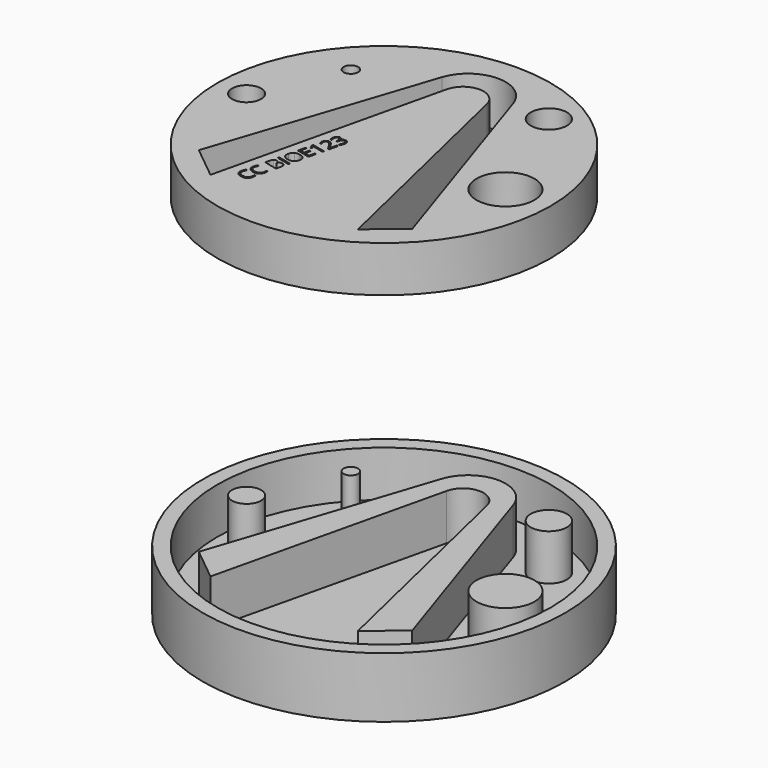
from build123d import *

# Parameters (mm, degrees)
F0_R     = 23
F1_DEPTH = 2
F3_R     = 2
F3_R_2   = 4
F3_R_3   = 1
F3_R_4   = 2.5
F4_DEPTH = 6.35
F0_R_2   = 25
F5_DEPTH = 8.35
F6_R     = 23
F6_R_2   = 2
F6_R_3   = 1
F6_R_4   = 4
F6_R_5   = 2.5
F7_DEPTH = 6.35


# Not quite as in the source:
# - a feature names something its author has since deleted; it is built from what else it names


with BuildPart() as f1:
    # F0 (on Top) → F1 (new body)
    with BuildSketch(Plane.XY):
        Circle(F0_R)
    extrude(amount=F1_DEPTH)

    # F3 (on face) → F4 (join)
    with BuildSketch(Plane.XY.offset(2)):
        with BuildLine():
            Line((14.693104138, -13.4988571827), (4.888704138, 16.1648631611))
            ThreePointArc((4.888704138, 16.1648631611), (-0.032147931, 19.721101458), (-4.953, 16.1648631611))
            Line((-4.953, 16.1648631611), (-14.7574, -13.4988571827))
            Line((-14.7574, -13.4988571827), (-10.182928455, -17.2135983478))
            Line((-10.182928455, -17.2135983478), (-2.7686, 14.2851547342))
            ThreePointArc((-2.7686, 14.2851547342), (-0.0045905534, 16.4740974526), (2.7594188933, 14.2851547342))
            Line((2.7594188933, 14.2851547342), (10.1737473482, -17.2135983478))
            Line((10.1737473482, -17.2135983478), (14.693104138, -13.4988571827))
        make_face()
        with Locations((-18.9738, 0)):
            Circle(F3_R)
        with Locations((16.764, 0)):
            Circle(F3_R_2)
        with Locations((-13.716, 11.43)):
            Circle(F3_R_3)
        with Locations((10.16, 15.748)):
            Circle(F3_R_4)
    extrude(amount=F4_DEPTH)

    # F0 (on Top) → F5 (join)
    with BuildSketch(Plane.XY):
        Circle(F0_R_2)
        Circle(F0_R, mode=Mode.SUBTRACT)
    extrude(amount=F5_DEPTH)


with BuildPart() as f7:
    # F6 (on offset) → F7 (new body)
    with BuildSketch(Plane.XY.offset(50.8)):
        Circle(F6_R)
        with BuildLine():
            add(Edge.make_bspline(
                [(-7.7742172335, -13.9858252735), (-7.9195629499, -14.1696054685), (-7.9681992906, -14.3761575918)],
                knots=[0, 0, 0, 1, 1, 1], degree=2))
            add(Edge.make_bspline(
                [(-7.9681992906, -14.3761575918), (-8.038764155, -14.6758372619), (-7.8800349733, -14.8963533518)],
                knots=[0, 0, 0, 1, 1, 1], degree=2))
            add(Edge.make_bspline(
                [(-7.8800349733, -14.8963533518), (-7.7213057917, -15.1168694417), (-7.3742663861, -15.198585991)],
                knots=[0, 0, 0, 1, 1, 1], degree=2))
            add(Edge.make_bspline(
                [(-7.3742663861, -15.198585991), (-7.0176754372, -15.2825516198), (-6.7834580083, -15.1610724694)],
                knots=[0, 0, 0, 1, 1, 1], degree=2))
            add(Edge.make_bspline(
                [(-6.7834580083, -15.1610724694), (-6.5492405793, -15.039593319), (-6.476332924, -14.7299641245)],
                knots=[0, 0, 0, 1, 1, 1], degree=2))
            add(Edge.make_bspline(
                [(-6.476332924, -14.7299641245), (-6.4315387605, -14.539729221), (-6.4425462525, -14.2796484846)],
                knots=[0, 0, 0, 1, 1, 1], degree=2))
            Line((-6.4425462525, -14.2796484846), (-6.2574851015, -14.3232243969))
            add(Edge.make_bspline(
                [(-6.2574851015, -14.3232243969), (-6.2307595366, -14.5290397409), (-6.2960765491, -14.8064324768)],
                knots=[0, 0, 0, 1, 1, 1], degree=2))
            add(Edge.make_bspline(
                [(-6.2960765491, -14.8064324768), (-6.390631593, -15.2079952752), (-6.6859947616, -15.3688426023)],
                knots=[0, 0, 0, 1, 1, 1], degree=2))
            add(Edge.make_bspline(
                [(-6.6859947616, -15.3688426023), (-6.9813579301, -15.5296899294), (-7.430280464, -15.4239832004)],
                knots=[0, 0, 0, 1, 1, 1], degree=2))
            add(Edge.make_bspline(
                [(-7.430280464, -15.4239832004), (-7.7112550286, -15.3578227831), (-7.8978430508, -15.2029949267)],
                knots=[0, 0, 0, 1, 1, 1], degree=2))
            add(Edge.make_bspline(
                [(-7.8978430508, -15.2029949267), (-8.0844310729, -15.0481670703), (-8.1521353496, -14.8228314606)],
                knots=[0, 0, 0, 1, 1, 1], degree=2))
            add(Edge.make_bspline(
                [(-8.1521353496, -14.8228314606), (-8.2198396262, -14.5974958509), (-8.1565842698, -14.3288586963)],
                knots=[0, 0, 0, 1, 1, 1], degree=2))
            add(Edge.make_bspline(
                [(-8.1565842698, -14.3288586963), (-8.0892993128, -14.0431083601), (-7.9346114369, -13.8535470478)],
                knots=[0, 0, 0, 1, 1, 1], degree=2))
            Line((-7.9346114369, -13.8535470478), (-7.7742172335, -13.9858252735))
        make_face(mode=Mode.SUBTRACT)
        with BuildLine():
            add(Edge.make_bspline(
                [(-7.3958096344, -12.3787781178), (-7.5411553508, -12.5625583127), (-7.5897916916, -12.769110436)],
                knots=[0, 0, 0, 1, 1, 1], degree=2))
            add(Edge.make_bspline(
                [(-7.5897916916, -12.769110436), (-7.6603565559, -13.0687901062), (-7.5016273743, -13.2893061961)],
                knots=[0, 0, 0, 1, 1, 1], degree=2))
            add(Edge.make_bspline(
                [(-7.5016273743, -13.2893061961), (-7.3428981926, -13.5098222859), (-6.995858787, -13.5915388353)],
                knots=[0, 0, 0, 1, 1, 1], degree=2))
            add(Edge.make_bspline(
                [(-6.995858787, -13.5915388353), (-6.6392678382, -13.675504464), (-6.4050504092, -13.5540253136)],
                knots=[0, 0, 0, 1, 1, 1], degree=2))
            add(Edge.make_bspline(
                [(-6.4050504092, -13.5540253136), (-6.1708329803, -13.4325461633), (-6.097925325, -13.1229169688)],
                knots=[0, 0, 0, 1, 1, 1], degree=2))
            add(Edge.make_bspline(
                [(-6.097925325, -13.1229169688), (-6.0531311614, -12.9326820653), (-6.0641386534, -12.6726013289)],
                knots=[0, 0, 0, 1, 1, 1], degree=2))
            Line((-6.0641386534, -12.6726013289), (-5.8790775025, -12.7161772411))
            add(Edge.make_bspline(
                [(-5.8790775025, -12.7161772411), (-5.8523519375, -12.9219925852), (-5.91766895, -13.1993853211)],
                knots=[0, 0, 0, 1, 1, 1], degree=2))
            add(Edge.make_bspline(
                [(-5.91766895, -13.1993853211), (-6.012223994, -13.6009481195), (-6.3075871625, -13.7617954466)],
                knots=[0, 0, 0, 1, 1, 1], degree=2))
            add(Edge.make_bspline(
                [(-6.3075871625, -13.7617954466), (-6.602950331, -13.9226427736), (-7.0518728649, -13.8169360446)],
                knots=[0, 0, 0, 1, 1, 1], degree=2))
            add(Edge.make_bspline(
                [(-7.0518728649, -13.8169360446), (-7.3328474295, -13.7507756274), (-7.5194354517, -13.5959477709)],
                knots=[0, 0, 0, 1, 1, 1], degree=2))
            add(Edge.make_bspline(
                [(-7.5194354517, -13.5959477709), (-7.7060234739, -13.4411199145), (-7.7737277505, -13.2157843049)],
                knots=[0, 0, 0, 1, 1, 1], degree=2))
            add(Edge.make_bspline(
                [(-7.7737277505, -13.2157843049), (-7.8414320272, -12.9904486952), (-7.7781766707, -12.7218115406)],
                knots=[0, 0, 0, 1, 1, 1], degree=2))
            add(Edge.make_bspline(
                [(-7.7781766707, -12.7218115406), (-7.7108917138, -12.4360612044), (-7.5562038378, -12.2464998921)],
                knots=[0, 0, 0, 1, 1, 1], degree=2))
            Line((-7.5562038378, -12.2464998921), (-7.3958096344, -12.3787781178))
        make_face(mode=Mode.SUBTRACT)
        with BuildLine():
            Line((-5.5836387497, -11.6684184118), (-7.4020138004, -11.2402499324))
            Line((-7.4020138004, -11.2402499324), (-7.2810320742, -10.7264565005))
            add(Edge.make_bspline(
                [(-7.2810320742, -10.7264565005), (-7.1958481942, -10.364691799), (-7.0495035891, -10.2284021007)],
                knots=[0, 0, 0, 1, 1, 1], degree=2))
            add(Edge.make_bspline(
                [(-7.0495035891, -10.2284021007), (-6.903158984, -10.0921124023), (-6.6695441547, -10.1471211345)],
                knots=[0, 0, 0, 1, 1, 1], degree=2))
            add(Edge.make_bspline(
                [(-6.6695441547, -10.1471211345), (-6.5075659001, -10.1852617717), (-6.4237246103, -10.3001443341)],
                knots=[0, 0, 0, 1, 1, 1], degree=2))
            add(Edge.make_bspline(
                [(-6.4237246103, -10.3001443341), (-6.3398833206, -10.4150268965), (-6.349605368, -10.5954581261)],
                knots=[0, 0, 0, 1, 1, 1], degree=2))
            Line((-6.349605368, -10.5954581261), (-6.337267958, -10.598363187))
            add(Edge.make_bspline(
                [(-6.337267958, -10.598363187), (-6.1688735289, -10.2007456693), (-5.8043229607, -10.2865855308)],
                knots=[0, 0, 0, 1, 1, 1], degree=2))
            add(Edge.make_bspline(
                [(-5.8043229607, -10.2865855308), (-5.5607586072, -10.3439370539), (-5.4626497723, -10.5409379793)],
                knots=[0, 0, 0, 1, 1, 1], degree=2))
            add(Edge.make_bspline(
                [(-5.4626497723, -10.5409379793), (-5.3645409373, -10.7379389046), (-5.4342623969, -11.0340367461)],
                knots=[0, 0, 0, 1, 1, 1], degree=2))
            Line((-5.4342623969, -11.0340367461), (-5.5836387497, -11.6684184118))
        make_face(mode=Mode.SUBTRACT)
        Polygon((-5.1452557016, -9.8066634355), (-5.195016582, -10.0179913304), (-7.0133916326, -9.5898228509), (-6.9636307522, -9.378494956), align=None, mode=Mode.SUBTRACT)
        with BuildLine():
            add(Edge.make_bspline(
                [(-6.3062887675, -7.5733382878), (-6.0057281249, -7.411824586), (-5.5679490583, -7.5149073891)],
                knots=[0, 0, 0, 1, 1, 1], degree=2))
            add(Edge.make_bspline(
                [(-5.5679490583, -7.5149073891), (-5.1313639345, -7.6177090573), (-4.9332428548, -7.8974862608)],
                knots=[0, 0, 0, 1, 1, 1], degree=2))
            add(Edge.make_bspline(
                [(-4.9332428548, -7.8974862608), (-4.735121775, -8.1772634642), (-4.8276151629, -8.5700706813)],
                knots=[0, 0, 0, 1, 1, 1], degree=2))
            add(Edge.make_bspline(
                [(-4.8276151629, -8.5700706813), (-4.9221702069, -8.9716334798), (-5.2193242898, -9.1320591044)],
                knots=[0, 0, 0, 1, 1, 1], degree=2))
            add(Edge.make_bspline(
                [(-5.2193242898, -9.1320591044), (-5.5164783727, -9.2924847291), (-5.9642069636, -9.187059135)],
                knots=[0, 0, 0, 1, 1, 1], degree=2))
            add(Edge.make_bspline(
                [(-5.9642069636, -9.187059135), (-6.4083537258, -9.0824769457), (-6.6011726397, -8.8060484659)],
                knots=[0, 0, 0, 1, 1, 1], degree=2))
            add(Edge.make_bspline(
                [(-6.6011726397, -8.8060484659), (-6.7939915535, -8.5296199861), (-6.6991553747, -8.1268632447)],
                knots=[0, 0, 0, 1, 1, 1], degree=2))
            add(Edge.make_bspline(
                [(-6.6991553747, -8.1268632447), (-6.60684941, -7.7348519895), (-6.3062887675, -7.5733382878)],
                knots=[0, 0, 0, 1, 1, 1], degree=2))
        make_face(mode=Mode.SUBTRACT)
        Polygon((-4.5111336235, -6.2662855689), (-4.3220926629, -6.3107985975), (-4.5607762079, -7.3244561274), (-6.3791512586, -6.8962876479), (-6.1404677136, -5.882630118), (-5.9526206958, -5.9268620117), (-6.1415433605, -6.7291916467), (-5.555715373, -6.8671351796), (-5.3782255284, -6.1133592229), (-5.1915724536, -6.1573099817), (-5.3690622982, -6.9110859383), (-4.7000562881, -7.0686152038), align=None, mode=Mode.SUBTRACT)
        with BuildLine():
            Line((-5.8951306421, -4.8407159393), (-4.0767555915, -5.2688844188))
            Line((-4.0767555915, -5.2688844188), (-4.1241736809, -5.4702627894))
            Line((-4.1241736809, -5.4702627894), (-5.4199997183, -5.1651376922))
            add(Edge.make_bspline(
                [(-5.4199997183, -5.1651376922), (-5.581977973, -5.1269970551), (-5.7237042931, -5.0831239174)],
                knots=[0, 0, 0, 1, 1, 1], degree=2))
            add(Edge.make_bspline(
                [(-5.7237042931, -5.0831239174), (-5.7035288056, -5.1151776487), (-5.6827106649, -5.1543134799)],
                knots=[0, 0, 0, 1, 1, 1], degree=2))
            add(Edge.make_bspline(
                [(-5.6827106649, -5.1543134799), (-5.6618925241, -5.1934493111), (-5.5098158676, -5.507329575)],
                knots=[0, 0, 0, 1, 1, 1], degree=2))
            Line((-5.5098158676, -5.507329575), (-5.6772677936, -5.5834129981))
            Line((-5.6772677936, -5.5834129981), (-5.9360826285, -5.0146336231))
            Line((-5.9360826285, -5.0146336231), (-5.8951306421, -4.8407159393))
        make_face(mode=Mode.SUBTRACT)
        with BuildLine():
            Line((-3.8238975565, -3.3369813429), (-3.6324687101, -3.3820566413))
            Line((-3.6324687101, -3.3820566413), (-3.9138847626, -4.5771934934))
            Line((-3.9138847626, -4.5771934934), (-4.091782256, -4.5353043907))
            Line((-4.091782256, -4.5353043907), (-4.4602061465, -3.9432359123))
            add(Edge.make_bspline(
                [(-4.4602061465, -3.9432359123), (-4.6303401451, -3.6721489959), (-4.7084610885, -3.5802458119)],
                knots=[0, 0, 0, 1, 1, 1], degree=2))
            add(Edge.make_bspline(
                [(-4.7084610885, -3.5802458119), (-4.786582032, -3.4883426279), (-4.8679279817, -3.4324341743)],
                knots=[0, 0, 0, 1, 1, 1], degree=2))
            add(Edge.make_bspline(
                [(-4.8679279817, -3.4324341743), (-4.9492739315, -3.3765257206), (-5.0523510026, -3.352254406)],
                knots=[0, 0, 0, 1, 1, 1], degree=2))
            add(Edge.make_bspline(
                [(-5.0523510026, -3.352254406), (-5.1980120375, -3.3179559461), (-5.303983949, -3.3862534306)],
                knots=[0, 0, 0, 1, 1, 1], degree=2))
            add(Edge.make_bspline(
                [(-5.303983949, -3.3862534306), (-5.4099558604, -3.4545509151), (-5.4468782462, -3.6113554171)],
                knots=[0, 0, 0, 1, 1, 1], degree=2))
            add(Edge.make_bspline(
                [(-5.4468782462, -3.6113554171), (-5.4734923518, -3.7243820125), (-5.4599786086, -3.8346760539)],
                knots=[0, 0, 0, 1, 1, 1], degree=2))
            add(Edge.make_bspline(
                [(-5.4599786086, -3.8346760539), (-5.4464648654, -3.9449700953), (-5.3774015974, -4.0922869327)],
                knots=[0, 0, 0, 1, 1, 1], degree=2))
            Line((-5.3774015974, -4.0922869327), (-5.5436595804, -4.1686514907))
            add(Edge.make_bspline(
                [(-5.5436595804, -4.1686514907), (-5.6934675452, -3.8683268883), (-5.6237460857, -3.5722290468)],
                knots=[0, 0, 0, 1, 1, 1], degree=2))
            add(Edge.make_bspline(
                [(-5.6237460857, -3.5722290468), (-5.56339579, -3.3159293023), (-5.3980094564, -3.201345243)],
                knots=[0, 0, 0, 1, 1, 1], degree=2))
            add(Edge.make_bspline(
                [(-5.3980094564, -3.201345243), (-5.2326231227, -3.0867611837), (-5.0113457036, -3.1388648551)],
                knots=[0, 0, 0, 1, 1, 1], degree=2))
            add(Edge.make_bspline(
                [(-5.0113457036, -3.1388648551), (-4.8382239817, -3.1796294181), (-4.6919477096, -3.3165642214)],
                knots=[0, 0, 0, 1, 1, 1], degree=2))
            add(Edge.make_bspline(
                [(-4.6919477096, -3.3165642214), (-4.5456714374, -3.4534990246), (-4.3495831821, -3.7802628779)],
                knots=[0, 0, 0, 1, 1, 1], degree=2))
            Line((-4.3495831821, -3.7802628779), (-4.0540694329, -4.2698938307))
            Line((-4.0540694329, -4.2698938307), (-4.0441199086, -4.2722366217))
            Line((-4.0441199086, -4.2722366217), (-3.8238975565, -3.3369813429))
        make_face(mode=Mode.SUBTRACT)
        with BuildLine():
            add(Edge.make_bspline(
                [(-5.0633344275, -1.7354274359), (-4.9075696273, -1.6171076522), (-4.6962417324, -1.6668685326)],
                knots=[0, 0, 0, 1, 1, 1], degree=2))
            add(Edge.make_bspline(
                [(-4.6962417324, -1.6668685326), (-4.5219260677, -1.7079142305), (-4.4342935655, -1.8316703943)],
                knots=[0, 0, 0, 1, 1, 1], degree=2))
            add(Edge.make_bspline(
                [(-4.4342935655, -1.8316703943), (-4.3466610634, -1.9554265581), (-4.3514210898, -2.1433268885)],
                knots=[0, 0, 0, 1, 1, 1], degree=2))
            Line((-4.3514210898, -2.1433268885), (-4.3414715656, -2.1456696795))
            add(Edge.make_bspline(
                [(-4.3414715656, -2.1456696795), (-4.2628674581, -1.9331525376), (-4.1259553749, -1.8538684166)],
                knots=[0, 0, 0, 1, 1, 1], degree=2))
            add(Edge.make_bspline(
                [(-4.1259553749, -1.8538684166), (-3.9890432917, -1.7745842956), (-3.8075639695, -1.817316803)],
                knots=[0, 0, 0, 1, 1, 1], degree=2))
            add(Edge.make_bspline(
                [(-3.8075639695, -1.817316803), (-3.5476823963, -1.8785105034), (-3.4500444675, -2.0917823797)],
                knots=[0, 0, 0, 1, 1, 1], degree=2))
            add(Edge.make_bspline(
                [(-3.4500444675, -2.0917823797), (-3.3524065387, -2.305054256), (-3.4305620458, -2.6369703847)],
                knots=[0, 0, 0, 1, 1, 1], degree=2))
            add(Edge.make_bspline(
                [(-3.4305620458, -2.6369703847), (-3.4645793709, -2.7814374767), (-3.5147223834, -2.896274599)],
                knots=[0, 0, 0, 1, 1, 1], degree=2))
            add(Edge.make_bspline(
                [(-3.5147223834, -2.896274599), (-3.564865396, -3.0111117212), (-3.6460028943, -3.111299822)],
                knots=[0, 0, 0, 1, 1, 1], degree=2))
            Line((-3.6460028943, -3.111299822), (-3.8426054934, -3.0650062722))
            add(Edge.make_bspline(
                [(-3.8426054934, -3.0650062722), (-3.756269934, -2.9605815352), (-3.694337279, -2.8340288698)],
                knots=[0, 0, 0, 1, 1, 1], degree=2))
            add(Edge.make_bspline(
                [(-3.694337279, -2.8340288698), (-3.6324046241, -2.7074762043), (-3.6042911323, -2.5880819134)],
                knots=[0, 0, 0, 1, 1, 1], degree=2))
            add(Edge.make_bspline(
                [(-3.6042911323, -2.5880819134), (-3.4933365515, -2.1168724453), (-3.8626628914, -2.0299080441)],
                knots=[0, 0, 0, 1, 1, 1], degree=2))
            add(Edge.make_bspline(
                [(-3.8626628914, -2.0299080441), (-4.1937830582, -1.9519399603), (-4.316170459, -2.4717031068)],
                knots=[0, 0, 0, 1, 1, 1], degree=2))
            Line((-4.316170459, -2.4717031068), (-4.3583406967, -2.6507945431))
            Line((-4.3583406967, -2.6507945431), (-4.5358402092, -2.6089991521))
            Line((-4.5358402092, -2.6089991521), (-4.4931077017, -2.4275198299))
            add(Edge.make_bspline(
                [(-4.4931077017, -2.4275198299), (-4.4430656863, -2.214997992), (-4.507704308, -2.0685129921)],
                knots=[0, 0, 0, 1, 1, 1], degree=2))
            add(Edge.make_bspline(
                [(-4.507704308, -2.0685129921), (-4.5723429296, -1.9220279923), (-4.7390969559, -1.8827628154)],
                knots=[0, 0, 0, 1, 1, 1], degree=2))
            add(Edge.make_bspline(
                [(-4.7390969559, -1.8827628154), (-4.8720225998, -1.8514631279), (-4.9695437862, -1.9249008374)],
                knots=[0, 0, 0, 1, 1, 1], degree=2))
            add(Edge.make_bspline(
                [(-4.9695437862, -1.9249008374), (-5.0670649726, -1.9983385469), (-5.1039873584, -2.1551430489)],
                knots=[0, 0, 0, 1, 1, 1], degree=2))
            add(Edge.make_bspline(
                [(-5.1039873584, -2.1551430489), (-5.1321008502, -2.2745373399), (-5.1245458414, -2.3878387859)],
                knots=[0, 0, 0, 1, 1, 1], degree=2))
            add(Edge.make_bspline(
                [(-5.1245458414, -2.3878387859), (-5.1169908325, -2.501140232), (-5.0617886691, -2.6573745916)],
                knots=[0, 0, 0, 1, 1, 1], degree=2))
            Line((-5.0617886691, -2.6573745916), (-5.225634458, -2.728846532))
            add(Edge.make_bspline(
                [(-5.225634458, -2.728846532), (-5.2876532627, -2.5962098956), (-5.3036056837, -2.4382963573)],
                knots=[0, 0, 0, 1, 1, 1], degree=2))
            add(Edge.make_bspline(
                [(-5.3036056837, -2.4382963573), (-5.3195581048, -2.2803828191), (-5.2814174677, -2.1184045644)],
                knots=[0, 0, 0, 1, 1, 1], degree=2))
            add(Edge.make_bspline(
                [(-5.2814174677, -2.1184045644), (-5.2190992276, -1.8537472196), (-5.0633344275, -1.7354274359)],
                knots=[0, 0, 0, 1, 1, 1], degree=2))
        make_face(mode=Mode.SUBTRACT)
        with Locations((-18.9738, 0)):
            Circle(F6_R_2, mode=Mode.SUBTRACT)
        with Locations((-13.716, 11.43)):
            Circle(F6_R_3, mode=Mode.SUBTRACT)
        with BuildLine():
            ThreePointArc((-4.953, 16.1648631611), (-0.032242339, 19.7210332305), (4.8885153219, 16.1648631611))
            Line((4.8885153219, 16.1648631611), (14.6929153219, -13.4988571827))
            Line((14.6929153219, -13.4988571827), (10.1761167759, -17.2121360336))
            Line((10.1761167759, -17.2121360336), (2.7593167759, 14.2860351819))
            ThreePointArc((2.7593167759, 14.2860351819), (-0.004641612, 16.4747610227), (-2.7686, 14.2860351819))
            Line((-2.7686, 14.2860351819), (-10.1854, -17.2121360336))
            Line((-10.1854, -17.2121360336), (-14.7574, -13.4988571827))
            Line((-14.7574, -13.4988571827), (-4.953, 16.1648631611))
        make_face(mode=Mode.SUBTRACT)
        with Locations((16.764, 0)):
            Circle(F6_R_4, mode=Mode.SUBTRACT)
        with Locations((10.16, 15.748)):
            Circle(F6_R_5, mode=Mode.SUBTRACT)
    extrude(amount=F7_DEPTH)


solid = Compound([f1.part, f7.part])
